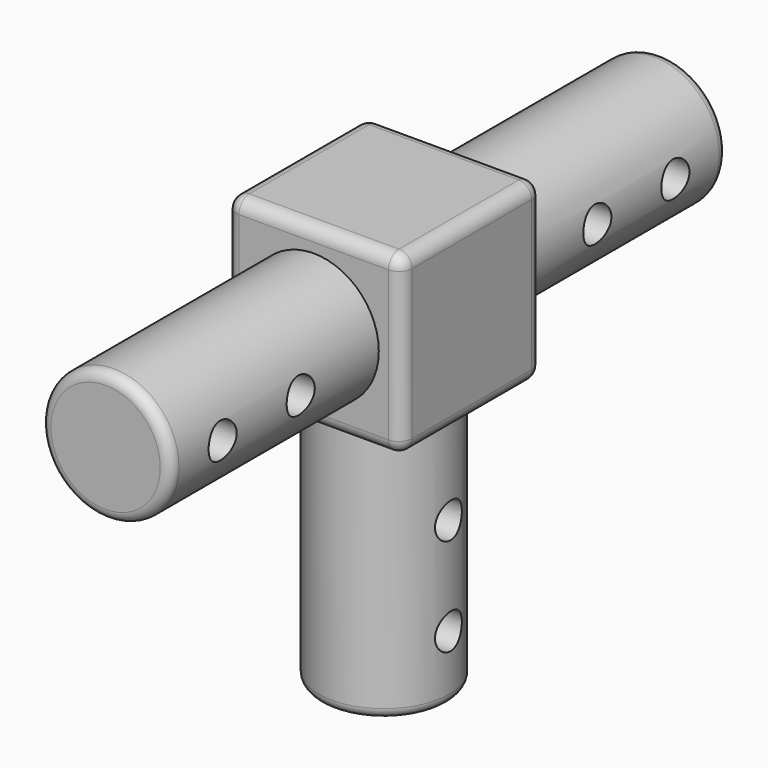
from build123d import *

# Parameters (mm, degrees)
F0_W      = 34.29
F0_H      = 34.29
F1_DEPTH  = 34.29
F2_R      = 12.7
F3_DEPTH  = 50.8
F4_R      = 3.429
F5_DEPTH  = 25.4
F6_R      = 3.429
F7_DEPTH  = 25.4
F8_R      = 3.429
F9_DEPTH  = 25.4
F10_R     = 2.54
F11_R     = 12.7
F12_DEPTH = 50.8
F13_R     = 3.429
F14_DEPTH = 25.4
F15_R     = 3.429
F16_DEPTH = 25.4
F17_R     = 12.7
F18_DEPTH = 50.8
F19_R     = 2.032
F20_R     = 3.429
F21_DEPTH = 25.4


with BuildPart() as f1:
    # F0 (on Top) → F1 (new body)
    with BuildSketch(Plane.XY):
        with Locations((3.6728888822, 6.5610635031)):
            Rectangle(F0_W, F0_H)
    extrude(amount=F1_DEPTH)

    # F2 (on face) → F3 (join)
    with BuildSketch(Plane.XZ.offset(10.5839364969)):
        with Locations((3.6728888822, 17.145)):
            Circle(F2_R)
    extrude(amount=F3_DEPTH)

    # F4 (on Front) → F5 (cut, symmetric)
    with BuildSketch(Plane.XZ):
        with Locations((3.6728888822, 53.34)):
            Circle(F4_R)
        with Locations((3.6728888822, 72.39)):
            Circle(F4_R)
    extrude(amount=F5_DEPTH, both=True, mode=Mode.SUBTRACT)

    # F6 (on Right) → F7 (cut, symmetric)
    with BuildSketch(Plane.YZ):
        with Locations((-29.6339364969, 17.145)):
            Circle(F6_R)
        with Locations((-48.6839364969, 17.145)):
            Circle(F6_R)
    extrude(amount=F7_DEPTH, both=True, mode=Mode.SUBTRACT)

    # F8 (on Front) → F9 (cut, symmetric)
    with BuildSketch(Plane.XZ):
        with Locations((-51.5721111178, 17.145)):
            Circle(F8_R)
        with Locations((-32.5221111178, 17.145)):
            Circle(F8_R)
    extrude(amount=F9_DEPTH, both=True, mode=Mode.SUBTRACT)

    # F10
    f10_edges = [f1.edges().sort_by_distance(p)[0] for p in [
        (20.817889, 23.706064, 17.145),
        (20.817889, 6.561064, 34.29),
        (20.817889, -10.583936, 17.145),
        (20.817889, 6.561064, 0),
        (3.672889, 23.706064, 0),
        (3.672889, 23.706064, 34.29),
        (-13.472111, 23.706064, 17.145),
        (-13.472111, 6.561064, 0),
        (3.672889, -10.583936, 0),
        (-13.472111, 6.561064, 34.29),
        (-13.472111, -10.583936, 17.145),
        (3.672889, -10.583936, 34.29),
    ]]
    fillet(f10_edges, radius=F10_R)

    # F11 (on face) → F12 (join)
    with BuildSketch(Plane(origin=(0, 23.7060635031, 0), x_dir=(-1, 0, 0), z_dir=(0, 1, 0))):
        with Locations((-3.6728888822, 17.145)):
            Circle(F11_R)
    extrude(amount=F12_DEPTH)

    # F13 (on Right) → F14 (cut, symmetric)
    with BuildSketch(Plane.YZ):
        with Locations((42.7560635031, 17.145)):
            Circle(F13_R)
        with Locations((61.8060635031, 17.145)):
            Circle(F13_R)
    extrude(amount=F14_DEPTH, both=True, mode=Mode.SUBTRACT)

    # F15 (on Front) → F16 (cut, symmetric)
    with BuildSketch(Plane.XZ):
        with Locations((58.9178888822, 17.145)):
            Circle(F15_R)
        with Locations((39.8678888822, 17.145)):
            Circle(F15_R)
    extrude(amount=F16_DEPTH, both=True, mode=Mode.SUBTRACT)

    # F17 (on face) → F18 (join)
    with BuildSketch(Plane(origin=(0, 0, 0), x_dir=(1, 0, 0), z_dir=(0, 0, -1))):
        with Locations((3.6728888822, -6.5610635031)):
            Circle(F17_R)
    extrude(amount=F18_DEPTH)

    # F19
    f19_edges = [f1.edges().sort_by_distance(p)[0] for p in [
        (-9.027111, -61.383936, 17.145),
        (16.372889, 74.506064, 17.145),
        (-9.027111, 6.561064, -50.8),
    ]]
    fillet(f19_edges, radius=F19_R)

    # F20 (on Right) → F21 (cut, symmetric)
    with BuildSketch(Plane.YZ):
        with Locations((7.0114927366, -19.05)):
            Circle(F20_R)
        with Locations((7.0114927366, -38.1)):
            Circle(F20_R)
    extrude(amount=F21_DEPTH, both=True, mode=Mode.SUBTRACT)


solid = f1.part
